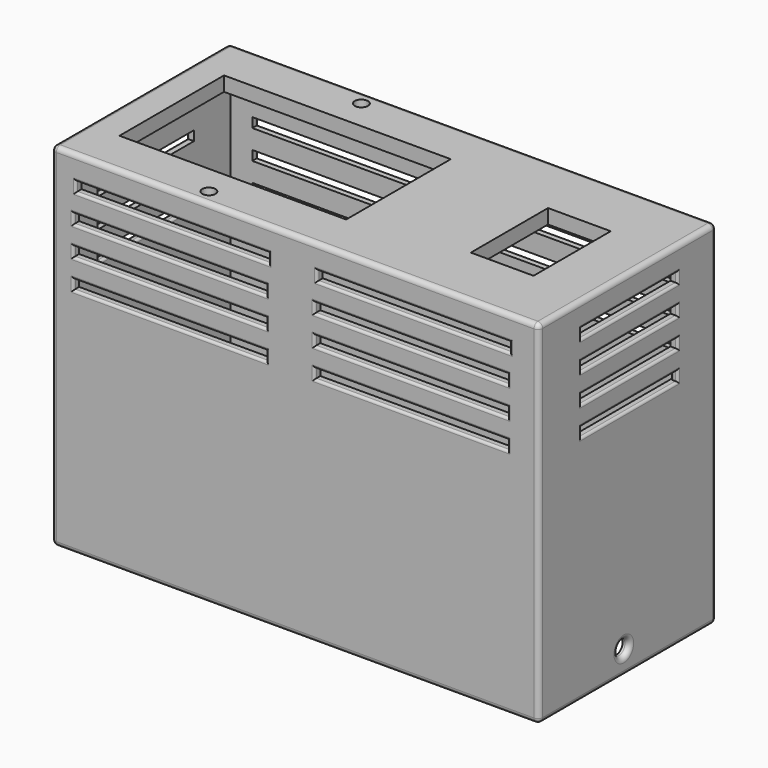
from build123d import *

# Parameters (mm, degrees)
F0_W          = 101
F0_H          = 46
F0_W_2        = 98
F0_H_2        = 43
F1_DEPTH      = 73
F0_R          = 1.375
F0_W_3        = 47
F0_H_3        = 27.1
F0_W_4        = 13
F0_H_4        = 20
F2_DEPTH      = 3
F4_R          = 1.55
F5_DEPTH      = 3
F6_R          = 1
F8_W          = 40
F8_H          = 2
F9_DEPTH      = 3
F7_W          = 40
F7_H          = 2
F10_DEPTH     = 3
F11_W         = 25
F11_H         = 2
F12_DEPTH     = 3
F13_W         = 25
F13_H         = 2
F14_DEPTH     = 3
F15_R         = 0.5
F16_TEXT_SIZE = 9.3799860527
F17_DEPTH     = 0.75


# Not quite as in the source:
# - Text() gives the source's letters only with a copy of the font that has no kerning and outlines rounded to 1/6400 em; it was checked with that copy


with BuildPart() as f1:
    # F0 (on Top) → F1 (new body)
    with BuildSketch(Plane.XY):
        Rectangle(F0_W, F0_H)
        Rectangle(F0_W_2, F0_H_2, mode=Mode.SUBTRACT)
    extrude(amount=-F1_DEPTH)

    # F0 (on Top) → F2 (join)
    with BuildSketch(Plane.XY):
        Rectangle(F0_W_2, F0_H_2)
        with Locations((-20.5, -19.75)):
            Circle(F0_R, mode=Mode.SUBTRACT)
        with Locations((-20.5, 0)):
            Rectangle(F0_W_3, F0_H_3, mode=Mode.SUBTRACT)
        with Locations((-20.5, 19.75)):
            Circle(F0_R, mode=Mode.SUBTRACT)
        with Locations((32.5, 0)):
            Rectangle(F0_W_4, F0_H_4, mode=Mode.SUBTRACT)
    extrude(amount=-F2_DEPTH)

    # F4 (on face) → F5 (cut)
    with BuildSketch(Plane.YZ.offset(50.5)):
        with Locations((-1, -68)):
            Circle(F4_R)
    extrude(amount=-F5_DEPTH, mode=Mode.SUBTRACT)

    # F6
    f6_edges = [f1.edges().sort_by_distance(p)[0] for p in [
        (0, -23, -73),
        (50.5, 0, -73),
        (0, 23, -73),
        (-50.5, 0, -73),
        (-50.5, -23, -36.5),
        (-50.5, 23, -36.5),
        (50.5, -23, -36.5),
        (50.5, 23, -36.5),
        (0, -23, 0),
        (50.5, 0, 0),
        (0, 23, 0),
        (-50.5, 0, 0),
        (50.5, -2.55, -68),
    ]]
    fillet(f6_edges, radius=F6_R)

    # F8 (on face) → F9 (cut)
    with BuildSketch(Plane(origin=(0, 23, 0), x_dir=(-1, 0, 0), z_dir=(0, 1, 0))):
        with Locations((24.5, -6)):
            Rectangle(F8_W, F8_H)
        with Locations((-25.5, -6)):
            Rectangle(F8_W, F8_H)
        with Locations((24.5, -12)):
            Rectangle(F8_W, F8_H)
        with Locations((-25.5, -12)):
            Rectangle(F8_W, F8_H)
        with Locations((24.5, -18)):
            Rectangle(F8_W, F8_H)
        with Locations((-25.5, -18)):
            Rectangle(F8_W, F8_H)
        with Locations((24.5, -24)):
            Rectangle(F8_W, F8_H)
        with Locations((-25.5, -24)):
            Rectangle(F8_W, F8_H)
    extrude(amount=-F9_DEPTH, mode=Mode.SUBTRACT)

    # F7 (on face) → F10 (cut)
    with BuildSketch(Plane.XZ.offset(23)):
        with Locations((24.5, -6)):
            Rectangle(F7_W, F7_H)
        with Locations((-25.5, -6)):
            Rectangle(F7_W, F7_H)
        with Locations((24, -12)):
            Rectangle(F7_W, F7_H)
        with Locations((-26, -12)):
            Rectangle(F7_W, F7_H)
        with Locations((24, -18)):
            Rectangle(F7_W, F7_H)
        with Locations((-26, -18)):
            Rectangle(F7_W, F7_H)
        with Locations((24, -24)):
            Rectangle(F7_W, F7_H)
        with Locations((-26, -24)):
            Rectangle(F7_W, F7_H)
    extrude(amount=-F10_DEPTH, mode=Mode.SUBTRACT)

    # F11 (on face) → F12 (cut)
    with BuildSketch(Plane.YZ.offset(50.5)):
        with Locations((0.5, -6)):
            Rectangle(F11_W, F11_H)
        with Locations((0.5, -12)):
            Rectangle(F11_W, F11_H)
        with Locations((0.5, -18)):
            Rectangle(F11_W, F11_H)
        with Locations((0.5, -24)):
            Rectangle(F11_W, F11_H)
    extrude(amount=-F12_DEPTH, mode=Mode.SUBTRACT)

    # F13 (on face) → F14 (cut)
    with BuildSketch(Plane(origin=(-50.5, 0, 0), x_dir=(0, -1, 0), z_dir=(-1, 0, 0))):
        with Locations((0.5, -6)):
            Rectangle(F13_W, F13_H)
        with Locations((0.5, -12)):
            Rectangle(F13_W, F13_H)
        with Locations((0.5, -18)):
            Rectangle(F13_W, F13_H)
        with Locations((0.5, -24)):
            Rectangle(F13_W, F13_H)
    extrude(amount=-F14_DEPTH, mode=Mode.SUBTRACT)

    # F15
    f15_edges = [f1.edges().sort_by_distance(p)[0] for p in [
        (44, -23, -24),
        (24, -23, -25),
        (24, -23, -23),
        (4, -23, -24),
        (24, -23, -19),
        (44, -23, -18),
        (24, -23, -17),
        (4, -23, -18),
        (4, -23, -12),
        (24, -23, -13),
        (44, -23, -12),
        (24, -23, -11),
        (24.5, -23, -7),
        (44.5, -23, -6),
        (24.5, -23, -5),
        (4.5, -23, -6),
        (-6, -23, -24),
        (-26, -23, -25),
        (-46, -23, -24),
        (-26, -23, -23),
        (-26, -23, -19),
        (-6, -23, -18),
        (-26, -23, -17),
        (-46, -23, -18),
        (-46, -23, -12),
        (-26, -23, -13),
        (-6, -23, -12),
        (-26, -23, -11),
        (-25.5, -23, -7),
        (-5.5, -23, -6),
        (-25.5, -23, -5),
        (-45.5, -23, -6),
        (50.5, 0.5, -25),
        (49, 13, -24),
        (50.5, 0.5, -23),
        (50.5, -12, -24),
        (50.5, -12, -18),
        (50.5, 0.5, -19),
        (50.5, 13, -18),
        (50.5, 0.5, -17),
        (50.5, 13, -12),
        (50.5, 0.5, -13),
        (50.5, 0.5, -11),
        (50.5, -12, -12),
        (50.5, -12, -6),
        (50.5, 0.5, -7),
        (50.5, 13, -6),
        (50.5, 0.5, -5),
        (50.5, 13, -24),
        (25.5, 23, -25),
        (5.5, 23, -24),
        (45.5, 23, -24),
        (25.5, 23, -23),
        (25.5, 23, -19),
        (45.5, 23, -18),
        (25.5, 23, -17),
        (5.5, 23, -18),
        (5.5, 23, -12),
        (25.5, 23, -13),
        (25.5, 23, -11),
        (45.5, 23, -12),
        (45.5, 23, -6),
        (25.5, 23, -7),
        (25.5, 23, -5),
        (5.5, 23, -6),
        (-4.5, 23, -24),
        (-24.5, 23, -25),
        (-44.5, 23, -24),
        (-24.5, 23, -23),
        (-24.5, 23, -19),
        (-44.5, 23, -18),
        (-24.5, 23, -17),
        (-4.5, 23, -18),
        (-4.5, 23, -12),
        (-24.5, 23, -13),
        (-24.5, 23, -11),
        (-44.5, 23, -12),
        (-44.5, 23, -6),
        (-24.5, 23, -7),
        (-24.5, 23, -5),
        (-4.5, 23, -6),
        (-50.5, -0.5, -5),
        (-50.5, -0.5, -7),
        (-50.5, 12, -6),
        (-50.5, -13, -6),
        (-50.5, -13, -12),
        (-50.5, -0.5, -13),
        (-50.5, -0.5, -11),
        (-50.5, 12, -12),
        (-50.5, -0.5, -17),
        (-50.5, 12, -18),
        (-50.5, -0.5, -19),
        (-50.5, -13, -18),
        (-50.5, -0.5, -23),
        (-49, -0.5, -25),
        (-50.5, 12, -24),
        (-50.5, -0.5, -25),
        (-50.5, -13, -24),
    ]]
    fillet(f15_edges, radius=F15_R)

    # F16 (on face) → F17 (cut)
    with BuildSketch(Plane(origin=(-50.5, 0, 0), x_dir=(0, -1, 0), z_dir=(-1, 0, 0))):
        with Locations((-6.9646397606, -39.2712727189)):
            Text('idk', F16_TEXT_SIZE, font='Open Sans', font_style=FontStyle.BOLD, text_align=(TextAlign.LEFT, TextAlign.BOTTOM))
    extrude(amount=-F17_DEPTH, mode=Mode.SUBTRACT)


solid = f1.part
